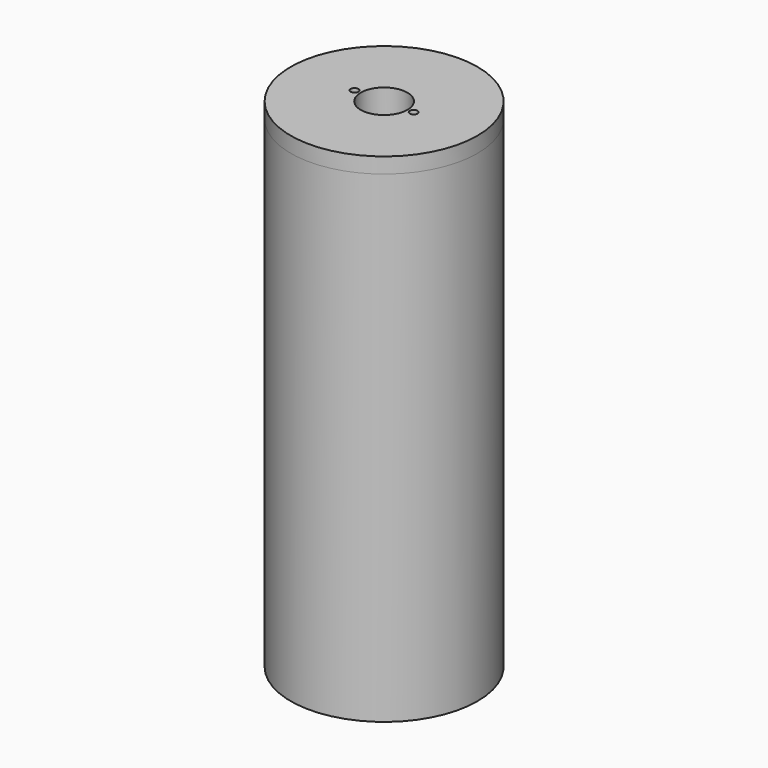
from build123d import *

# Parameters (mm, degrees)
F0_R     = 30
F0_R_2   = 25
F1_DEPTH = 155
F0_R_3   = 1.25
F0_R_4   = 7.5
F2_DEPTH = 10
F3_DEPTH = 5


with BuildPart() as f1:
    # F0 (on Top) → F1 (new body)
    with BuildSketch(Plane.XY):
        Circle(F0_R)
        Circle(F0_R_2, mode=Mode.SUBTRACT)
    extrude(amount=-F1_DEPTH)


with BuildPart() as f2:
    # F0 (on Top) → F2 (new body)
    with BuildSketch(Plane.XY):
        Circle(F0_R_2)
        with Locations((-9.5, 0)):
            Circle(F0_R_3, mode=Mode.SUBTRACT)
        Circle(F0_R_4, mode=Mode.SUBTRACT)
        with Locations((9.5, 0)):
            Circle(F0_R_3, mode=Mode.SUBTRACT)
    extrude(amount=-F2_DEPTH)

    # F0 (on Top) → F3 (join)
    with BuildSketch(Plane.XY):
        Circle(F0_R)
        Circle(F0_R_2, mode=Mode.SUBTRACT)
        Circle(F0_R_2)
        with Locations((-9.5, 0)):
            Circle(F0_R_3, mode=Mode.SUBTRACT)
        Circle(F0_R_4, mode=Mode.SUBTRACT)
        with Locations((9.5, 0)):
            Circle(F0_R_3, mode=Mode.SUBTRACT)
    extrude(amount=F3_DEPTH)


solid = Compound([f1.part, f2.part])
